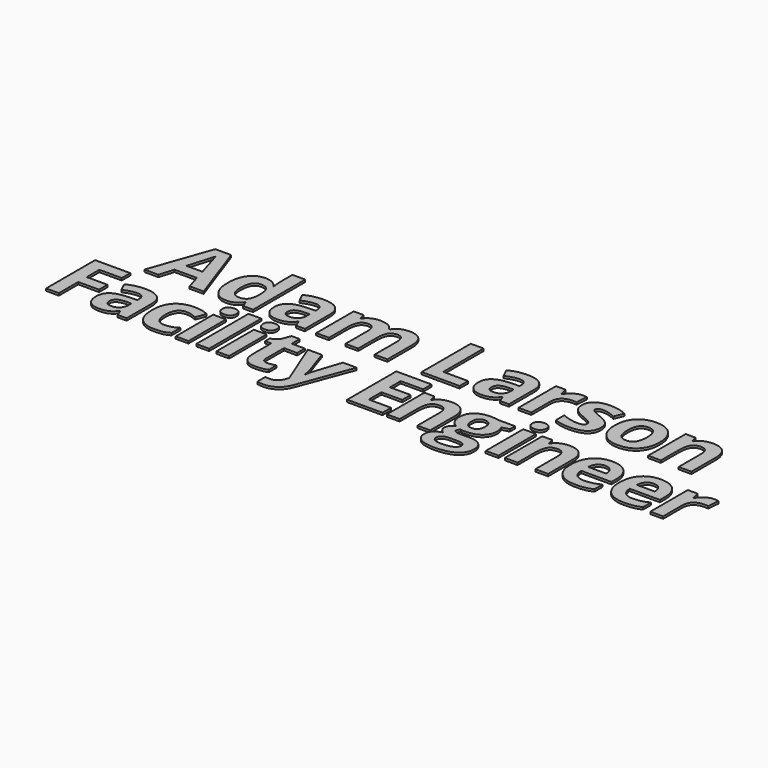
from build123d import *

# Parameters (mm, degrees)
F0_TEXT_SIZE = 24.6944444444
F1_DEPTH     = 0.635


# Not quite as in the source:
# - Text() gives the source's letters only with a copy of the font that has no kerning and outlines rounded to 1/6400 em; it was checked with that copy


with BuildPart() as f1:
    # F0 (on Top) → F1 (new body)
    with BuildSketch(Plane.XY):
        with Locations((-62.87042038, -48.5506180928)):
            Text('A', F0_TEXT_SIZE, font='Open Sans', font_style=FontStyle.BOLD, text_align=(TextAlign.LEFT, TextAlign.BOTTOM))
        with Locations((-45.3304746335, -48.5506180928)):
            Text('d', F0_TEXT_SIZE, font='Open Sans', font_style=FontStyle.BOLD, text_align=(TextAlign.LEFT, TextAlign.BOTTOM))
        with Locations((-29.7644307966, -48.5506180928)):
            Text('a', F0_TEXT_SIZE, font='Open Sans', font_style=FontStyle.BOLD, text_align=(TextAlign.LEFT, TextAlign.BOTTOM))
        with Locations((-15.3870827064, -48.5506180928)):
            Text('m', F0_TEXT_SIZE, font='Open Sans', font_style=FontStyle.BOLD, text_align=(TextAlign.LEFT, TextAlign.BOTTOM))
        with Locations((14.6604889082, -48.5506180928)):
            Text('L', F0_TEXT_SIZE, font='Open Sans', font_style=FontStyle.BOLD, text_align=(TextAlign.LEFT, TextAlign.BOTTOM))
        with Locations((28.9095692034, -48.5506180928)):
            Text('a', F0_TEXT_SIZE, font='Open Sans', font_style=FontStyle.BOLD, text_align=(TextAlign.LEFT, TextAlign.BOTTOM))
        with Locations((42.7902723284, -48.5506180928)):
            Text('r', F0_TEXT_SIZE, font='Open Sans', font_style=FontStyle.BOLD, text_align=(TextAlign.LEFT, TextAlign.BOTTOM))
        with Locations((53.900016252, -48.5506180928)):
            Text('s', F0_TEXT_SIZE, font='Open Sans', font_style=FontStyle.BOLD, text_align=(TextAlign.LEFT, TextAlign.BOTTOM))
        with Locations((65.8131564429, -48.5506180928)):
            Text('o', F0_TEXT_SIZE, font='Open Sans', font_style=FontStyle.BOLD, text_align=(TextAlign.LEFT, TextAlign.BOTTOM))
        with Locations((-76.58642038, -69.5056180928)):
            Text('F', F0_TEXT_SIZE, font='Open Sans', font_style=FontStyle.BOLD, text_align=(TextAlign.LEFT, TextAlign.BOTTOM))
        with Locations((-64.2529785397, -69.5056180928)):
            Text('a', F0_TEXT_SIZE, font='Open Sans', font_style=FontStyle.BOLD, text_align=(TextAlign.LEFT, TextAlign.BOTTOM))
        with Locations((-50.3527072723, -69.5056180928)):
            Text('c', F0_TEXT_SIZE, font='Open Sans', font_style=FontStyle.BOLD, text_align=(TextAlign.LEFT, TextAlign.BOTTOM))
        with Locations((-39.0224772376, -69.5056180928)):
            Text('i', F0_TEXT_SIZE, font='Open Sans', font_style=FontStyle.BOLD, text_align=(TextAlign.LEFT, TextAlign.BOTTOM))
        with Locations((-33.0955900848, -69.5056180928)):
            Text('l', F0_TEXT_SIZE, font='Open Sans', font_style=FontStyle.BOLD, text_align=(TextAlign.LEFT, TextAlign.BOTTOM))
        with Locations((-27.3384772376, -69.5056180928)):
            Text('i', F0_TEXT_SIZE, font='Open Sans', font_style=FontStyle.BOLD, text_align=(TextAlign.LEFT, TextAlign.BOTTOM))
        with Locations((-20.5224247203, -69.5056180928)):
            Text('t', F0_TEXT_SIZE, font='Open Sans', font_style=FontStyle.BOLD, text_align=(TextAlign.LEFT, TextAlign.BOTTOM))
        with Locations((-9.8847966821, -69.5056180928)):
            Text('y', F0_TEXT_SIZE, font='Open Sans', font_style=FontStyle.BOLD, text_align=(TextAlign.LEFT, TextAlign.BOTTOM))
        with Locations((80.0676937693, -48.5506180928)):
            Text('n', F0_TEXT_SIZE, font='Open Sans', font_style=FontStyle.BOLD, text_align=(TextAlign.LEFT, TextAlign.BOTTOM))
        with Locations((10.0044285784, -69.5056180928)):
            Text('E', F0_TEXT_SIZE, font='Open Sans', font_style=FontStyle.BOLD, text_align=(TextAlign.LEFT, TextAlign.BOTTOM))
        with Locations((21.7031460263, -69.5056180928)):
            Text('n', F0_TEXT_SIZE, font='Open Sans', font_style=FontStyle.BOLD, text_align=(TextAlign.LEFT, TextAlign.BOTTOM))
        with Locations((36.0281286652, -69.5056180928)):
            Text('g', F0_TEXT_SIZE, font='Open Sans', font_style=FontStyle.BOLD, text_align=(TextAlign.LEFT, TextAlign.BOTTOM))
        with Locations((50.1315227624, -69.5056180928)):
            Text('i', F0_TEXT_SIZE, font='Open Sans', font_style=FontStyle.BOLD, text_align=(TextAlign.LEFT, TextAlign.BOTTOM))
        with Locations((55.6121460263, -69.5056180928)):
            Text('n', F0_TEXT_SIZE, font='Open Sans', font_style=FontStyle.BOLD, text_align=(TextAlign.LEFT, TextAlign.BOTTOM))
        with Locations((70.0046525367, -69.5056180928)):
            Text('e', F0_TEXT_SIZE, font='Open Sans', font_style=FontStyle.BOLD, text_align=(TextAlign.LEFT, TextAlign.BOTTOM))
        with Locations((83.9746525367, -69.5056180928)):
            Text('e', F0_TEXT_SIZE, font='Open Sans', font_style=FontStyle.BOLD, text_align=(TextAlign.LEFT, TextAlign.BOTTOM))
        with Locations((97.4557245853, -69.5056180928)):
            Text('r', F0_TEXT_SIZE, font='Open Sans', font_style=FontStyle.BOLD, text_align=(TextAlign.LEFT, TextAlign.BOTTOM))
    extrude(amount=F1_DEPTH)


solid = f1.part
